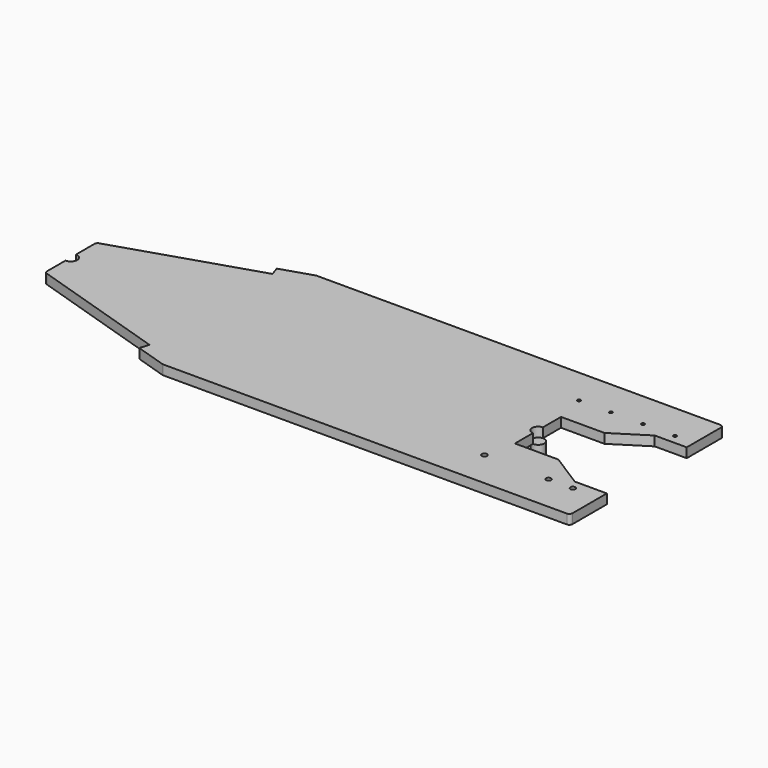
from build123d import *

# Parameters (mm, degrees)
F0_R     = 4
F0_R_2   = 2.5
F1_DEPTH = 15
F2_R     = 5
F3_R     = 5
F4_R     = 5
F5_R     = 10.2639763847
F5_R_2   = 9.6795888004
F6_DEPTH = 25
F7_DEPTH = 25


# Not quite as in the source:
# - a feature names something its author has since deleted; it is built from what else it names


with BuildPart() as f1:
    # F0 (on Top) → F1 (new body)
    with BuildSketch(Plane.XY):
        Polygon((0, 50), (0, 0), (0, -50), (219.0890230021, -120), (214.5238056108, -134.2884145436), (263.6986042887, -150), (900, -150), (900, -78), (850, -78), (797.8563520055, -45), (785, -45), (730, -45), (730, 45), (785, 45), (797.8563520055, 45), (850, 78), (900, 78), (900, 150), (263.6986042887, 150), (214.5238056108, 134.2884145436), (219.0890230021, 120), align=None)
        with Locations((720, -92)):
            Circle(F0_R, mode=Mode.SUBTRACT)
        with Locations((821, -93)):
            Circle(F0_R, mode=Mode.SUBTRACT)
        with Locations((859, -93)):
            Circle(F0_R, mode=Mode.SUBTRACT)
        with Locations((720, 92.5)):
            Circle(F0_R_2, mode=Mode.SUBTRACT)
        with Locations((770, 92.5)):
            Circle(F0_R_2, mode=Mode.SUBTRACT)
        with Locations((820, 92.5)):
            Circle(F0_R_2, mode=Mode.SUBTRACT)
        with Locations((870, 92.5)):
            Circle(F0_R_2, mode=Mode.SUBTRACT)
    extrude(amount=F1_DEPTH)

    # F2
    f2_edges = [f1.edges().sort_by_distance(p)[0] for p in [
        (263.698604, -150, 7.5),
    ]]
    fillet(f2_edges, radius=F2_R)

    # F3
    f3_edges = [f1.edges().sort_by_distance(p)[0] for p in [
        (0, -50, 7.5),
        (0, 50, 7.5),
    ]]
    fillet(f3_edges, radius=F3_R)

    # F4
    f4_edges = [f1.edges().sort_by_distance(p)[0] for p in [
        (900, 150, 7.5),
        (900, -150, 7.5),
    ]]
    fillet(f4_edges, radius=F4_R)

    # F5 (on Top) → F6 (cut)
    with BuildSketch(Plane.XY):
        Circle(F5_R)
        with Locations((730.375289917, 0)):
            Circle(F5_R_2)
    extrude(amount=F6_DEPTH, mode=Mode.SUBTRACT)

    # F5 (on Top) → F7 (join)
    with BuildSketch(Plane.XY):
        Circle(F5_R)
        with Locations((730.375289917, 0)):
            Circle(F5_R_2)
    extrude(amount=-F7_DEPTH)


solid = f1.part
